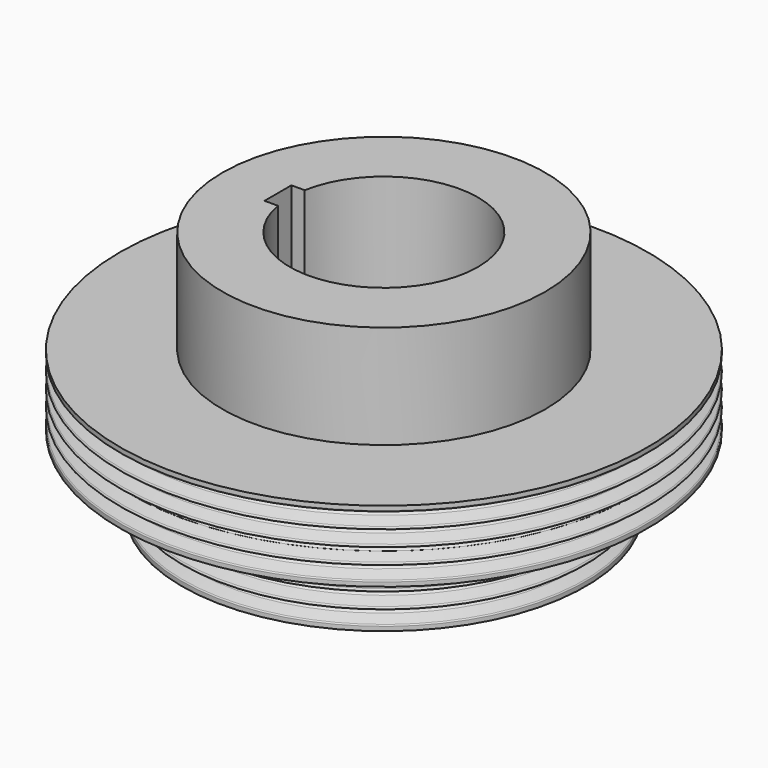
from build123d import *

# Parameters (mm, degrees)
F0_W     = 10
F0_H     = 15.38
F3_DEPTH = 36.6194192331


# Not quite as in the source:
# - a feature names something its author has since deleted; it is built from what else it names


with BuildPart() as f1:
    # F0 (on Front) → F1 (revolve)
    with BuildSketch(Plane.XZ):
        with BuildLine():
            Line((-30, 0), (-14, 0))
            Line((-14, 0), (-14, 10.6194192331))
            Line((-14, 10.6194192331), (-24, 10.6194192331))
            Line((-24, 10.6194192331), (-39.25, 10.6194192331))
            Line((-39.25, 10.6194192331), (-39.25, 9.9893224386))
            ThreePointArc((-39.25, 9.9893224386), (-39.2138304089, 9.8746071513), (-39.1184040287, 9.8013839144))
            Line((-39.1184040287, 9.8013839144), (-37.4531919427, 9.1952962814))
            ThreePointArc((-37.4531919427, 9.1952962814), (-37.19, 8.8194192331), (-37.4531919427, 8.4435421848))
            Line((-37.4531919427, 8.4435421848), (-39.1184040287, 7.8374545517))
            ThreePointArc((-39.1184040287, 7.8374545517), (-39.25, 7.6495160276), (-39.1184040287, 7.4615775034))
            Line((-39.1184040287, 7.4615775034), (-37.4531919427, 6.8554898704))
            ThreePointArc((-37.4531919427, 6.8554898704), (-37.19, 6.4796128221), (-37.4531919427, 6.1037357737))
            Line((-37.4531919427, 6.1037357737), (-39.1184040287, 5.4976481407))
            ThreePointArc((-39.1184040287, 5.4976481407), (-39.25, 5.3097096165), (-39.1184040287, 5.1217710924))
            Line((-39.1184040287, 5.1217710924), (-37.4531919427, 4.5156834593))
            ThreePointArc((-37.4531919427, 4.5156834593), (-37.2623391823, 4.3692369856), (-37.19, 4.139806411))
            ThreePointArc((-37.19, 4.139806411), (-37.2623391823, 3.9103758365), (-37.4531919427, 3.7639293627))
            Line((-37.4531919427, 3.7639293627), (-39.1184040287, 3.1578417297))
            ThreePointArc((-39.1184040287, 3.1578417297), (-39.25, 2.9699032055), (-39.1184040287, 2.7819646814))
            Line((-39.1184040287, 2.7819646814), (-37.4531919427, 2.1758770483))
            ThreePointArc((-37.4531919427, 2.1758770483), (-37.19, 1.8), (-37.4531919427, 1.4241229517))
            Line((-37.4531919427, 1.4241229517), (-39.1184040287, 0.8180353186))
            ThreePointArc((-39.1184040287, 0.8180353186), (-39.2138304089, 0.7448120818), (-39.25, 0.6300967945))
            Line((-39.25, 0.6300967945), (-39.25, 0))
            Line((-39.25, 0), (-30, 0))
        make_face()
        with Locations((-19, 18.3094192331)):
            Rectangle(F0_W, F0_H)
        with BuildLine():
            Line((-14, -10.62), (-14, 0))
            Line((-14, 0), (-30, 0))
            Line((-30, 0), (-30, -0.63))
            ThreePointArc((-30, -0.63), (-29.9638304089, -0.7447152873), (-29.8684040287, -0.8179385242))
            Line((-29.8684040287, -0.8179385242), (-28.202926002, -1.4241229517))
            ThreePointArc((-28.202926002, -1.4241229517), (-27.9397340593, -1.8), (-28.202926002, -2.1758770483))
            Line((-28.202926002, -2.1758770483), (-29.8684040287, -2.7820614758))
            ThreePointArc((-29.8684040287, -2.7820614758), (-30, -2.97), (-29.8684040287, -3.1579385242))
            Line((-29.8684040287, -3.1579385242), (-28.202926002, -3.7641229517))
            ThreePointArc((-28.202926002, -3.7641229517), (-27.9397340593, -4.14), (-28.202926002, -4.5158770483))
            Line((-28.202926002, -4.5158770483), (-29.8684040287, -5.1220614758))
            ThreePointArc((-29.8684040287, -5.1220614758), (-30, -5.31), (-29.8684040287, -5.4979385242))
            Line((-29.8684040287, -5.4979385242), (-28.202926002, -6.1041229517))
            ThreePointArc((-28.202926002, -6.1041229517), (-27.9397340593, -6.48), (-28.202926002, -6.8558770483))
            Line((-28.202926002, -6.8558770483), (-29.8684040287, -7.4620614758))
            ThreePointArc((-29.8684040287, -7.4620614758), (-30, -7.65), (-29.8684040287, -7.8379385242))
            Line((-29.8684040287, -7.8379385242), (-28.202926002, -8.4441229517))
            ThreePointArc((-28.202926002, -8.4441229517), (-27.9397340593, -8.82), (-28.202926002, -9.1958770483))
            Line((-28.202926002, -9.1958770483), (-29.8684040287, -9.8020614758))
            ThreePointArc((-29.8684040287, -9.8020614758), (-29.9638304089, -9.8752847127), (-30, -9.99))
            Line((-30, -9.99), (-30, -10.62))
            Line((-30, -10.62), (-14, -10.62))
        make_face()
    revolve(axis=Axis((0, 0, 5.3097096165), (0, 0, -1)))

    # F2 (on face) → F3 (cut, through all)
    with BuildSketch(Plane.XY.offset(25.9994192331)):
        with BuildLine():
            Line((-15.75, -2.5), (-13.774977314, -2.5))
            ThreePointArc((-13.774977314, -2.5), (-13.943630847, -1.2550533066), (-14, 0))
            Line((-14, 0), (-15.75, 0))
            Line((-15.75, 0), (-15.75, -2.5))
        make_face()
        with BuildLine():
            ThreePointArc((-14, 0), (-13.943630847, 1.2550533066), (-13.774977314, 2.5))
            Line((-13.774977314, 2.5), (-15.75, 2.5))
            Line((-15.75, 2.5), (-15.75, 0))
            Line((-15.75, 0), (-14, 0))
        make_face()
    extrude(amount=-F3_DEPTH, mode=Mode.SUBTRACT)


solid = f1.part
